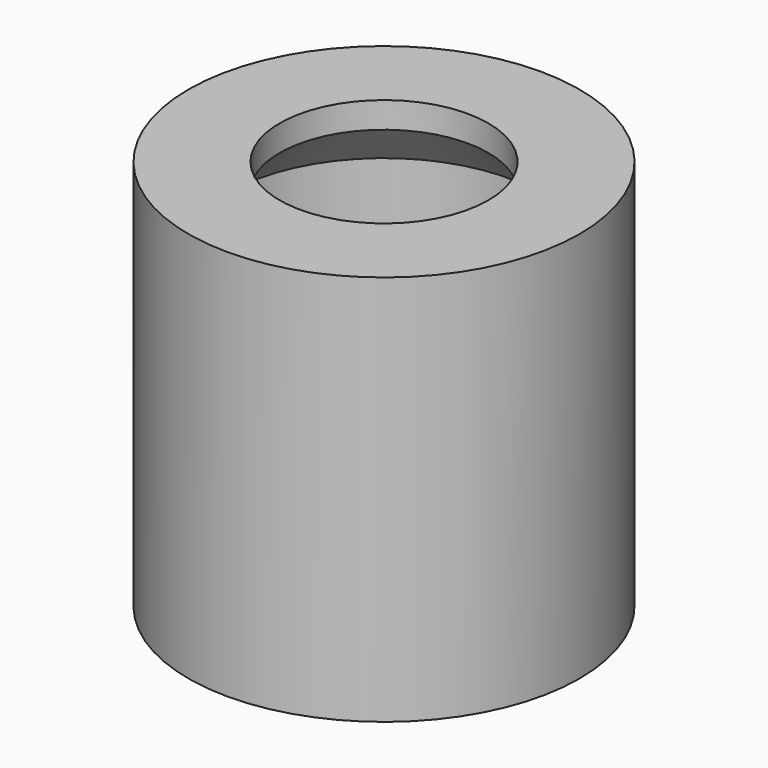
from build123d import *

# Parameters (mm, degrees)
F0_R     = 7.5
F0_R_2   = 4
F2_DEPTH = 15
F3_R     = 6
F4_DEPTH = 9
F5_SIZE  = 1.99999


# Not quite as in the source:
# - a fillet or chamfer is up to 0.001 mm smaller than in the source, because OpenCascade refuses the exact size


with BuildPart() as f2:
    # F0 (on Top) → F2 (new body)
    with BuildSketch(Plane.XY):
        Circle(F0_R)
        Circle(F0_R_2, mode=Mode.SUBTRACT)
    extrude(amount=-F2_DEPTH)

    # F3 (on offset) → F4 (cut)
    with BuildSketch(Plane.XY.offset(-3)):
        Circle(F3_R)
    extrude(amount=-F4_DEPTH, mode=Mode.SUBTRACT)

    # F5 (size 2 in the source; OpenCascade refuses exactly that, so slightly less here)
    f5_edges = [f2.edges().sort_by_distance(p)[0] for p in [
        (-4, 0, -3),
        (-4, 0, -12),
    ]]
    chamfer(f5_edges, length=F5_SIZE)


solid = f2.part
